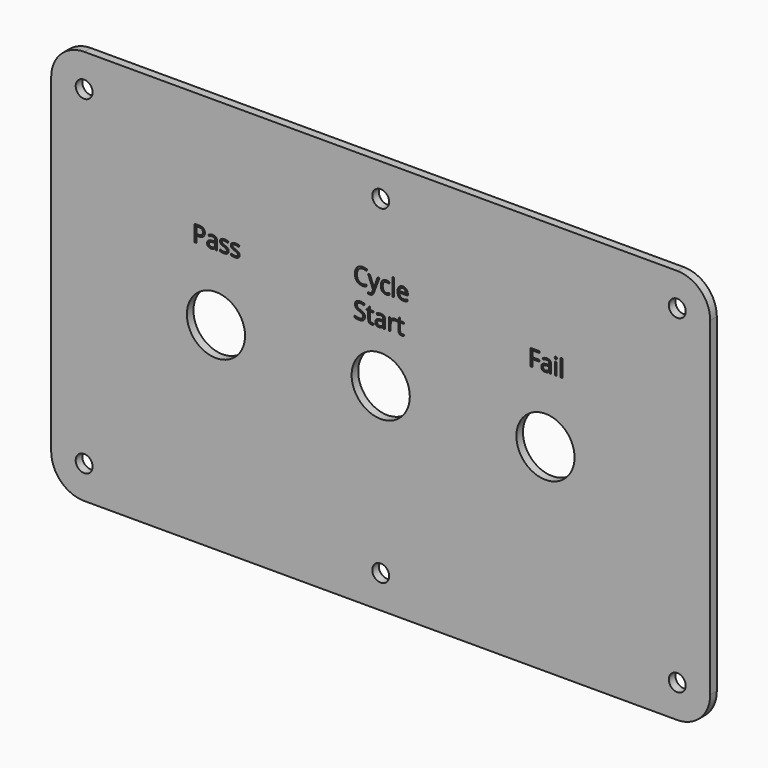
from build123d import *

# Parameters (mm, degrees)
F1_DEPTH     = 3.175
F2_R         = 11.2141
F3_DEPTH     = 25.4
F4_R         = 3.2639
F5_DEPTH     = 25.4
F6_TEXT_SIZE = 8.8194444444
F7_TEXT_SIZE = 8.8194444444
F8_TEXT_SIZE = 8.8194444444
F9_DEPTH     = 0.635


# Not quite as in the source:
# - Text() gives the source's letters only with a copy of the font that has no kerning and outlines rounded to 1/6400 em; it was checked with that copy


with BuildPart() as f1:
    # F0 (on Front) → F1 (new body)
    with BuildSketch(Plane.XZ):
        with BuildLine():
            Line((114.3, 76.2), (-114.3, 76.2))
            ThreePointArc((-114.3, 76.2), (-123.2802561211, 72.4802561211), (-127, 63.5))
            Line((-127, 63.5), (-127, -63.5))
            ThreePointArc((-127, -63.5), (-123.2802561211, -72.4802561211), (-114.3, -76.2))
            Line((-114.3, -76.2), (114.3, -76.2))
            ThreePointArc((114.3, -76.2), (123.2802561211, -72.4802561211), (127, -63.5))
            Line((127, -63.5), (127, 63.5))
            ThreePointArc((127, 63.5), (123.2802561211, 72.4802561211), (114.3, 76.2))
        make_face()
    extrude(amount=F1_DEPTH)

    # F2 (on face) → F3 (cut)
    with BuildSketch(Plane.XZ.offset(3.175)):
        with Locations((-63.5, 0)):
            Circle(F2_R)
        Circle(F2_R)
        with Locations((63.5, 0)):
            Circle(F2_R)
    extrude(amount=-F3_DEPTH, mode=Mode.SUBTRACT)

    # F4 (on face) → F5 (cut)
    with BuildSketch(Plane.XZ.offset(3.175)):
        with Locations((-114.3, 63.5)):
            Circle(F4_R)
        with Locations((-114.3, -63.5)):
            Circle(F4_R)
        with Locations((0, 63.5)):
            Circle(F4_R)
        with Locations((0, -63.5)):
            Circle(F4_R)
        with Locations((114.3, 63.5)):
            Circle(F4_R)
        with Locations((114.3, -63.5)):
            Circle(F4_R)
    extrude(amount=-F5_DEPTH, mode=Mode.SUBTRACT)

    # F6 (on face) + F7 (on face) + F8 (on face) → F9 (cut)
    with BuildSketch(Plane.XZ.offset(3.175)):
        with Locations((-72.6115885417, 25.4)):
            Text('Pass', F6_TEXT_SIZE, font='Open Sans', text_align=(TextAlign.LEFT, TextAlign.BOTTOM))
    with BuildSketch(Plane.XZ.offset(3.175)):
        with Locations((-10.4627549913, 31.75)):
            Text('Cycle', F7_TEXT_SIZE, font='Open Sans', text_align=(TextAlign.LEFT, TextAlign.BOTTOM))
        with Locations((-10.4627549913, 19.7555555556)):
            Text('Start', F7_TEXT_SIZE, font='Open Sans', text_align=(TextAlign.LEFT, TextAlign.BOTTOM))
    with BuildSketch(Plane.XZ.offset(3.175)):
        with Locations((56.9198676215, 25.4)):
            Text('Fail', F8_TEXT_SIZE, font='Open Sans', text_align=(TextAlign.LEFT, TextAlign.BOTTOM))
    extrude(amount=-F9_DEPTH, mode=Mode.SUBTRACT)


solid = f1.part
